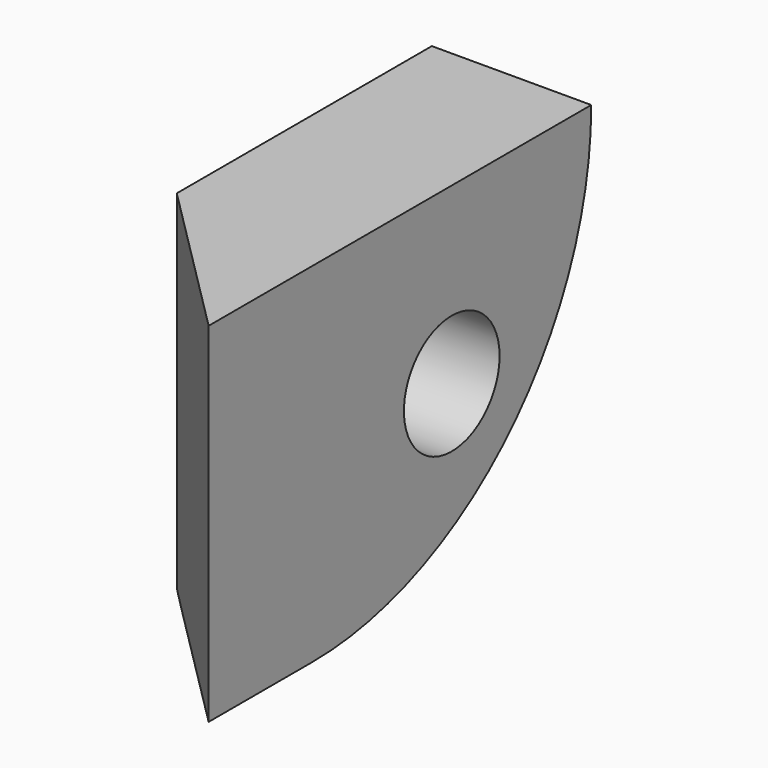
from build123d import *

# Parameters (mm, degrees)
F0_W     = 76.2
F0_H     = 55.5625
F1_DEPTH = 25.4
F2_R     = 55.56249
F3_R     = 9.525
F4_DEPTH = 25.4
F6_DEPTH = 55.5635


# Not quite as in the source:
# - a fillet or chamfer is up to 0.001 mm smaller than in the source, because OpenCascade refuses the exact size


with BuildPart() as f1:
    # F0 (on Right) → F1 (new body)
    with BuildSketch(Plane.YZ):
        Rectangle(F0_W, F0_H)
    extrude(amount=F1_DEPTH)

    # F2 (radius 55.5625 in the source; OpenCascade refuses exactly that, so slightly less here)
    f2_edges = [f1.edges().sort_by_distance(p)[0] for p in [
        (12.7, 38.1, -27.78125),
    ]]
    fillet(f2_edges, radius=F2_R)

    # F3 (on face) → F4 (cut)
    with BuildSketch(Plane.YZ.offset(25.4)):
        with Locations((10.31875, 0)):
            Circle(F3_R)
    extrude(amount=-F4_DEPTH, mode=Mode.SUBTRACT)

    # F5 (on face) → F6 (cut, through all)
    with BuildSketch(Plane.XY.offset(27.78125)):
        Polygon((0, -38.1), (25.4, -38.1), (0, -12.7), align=None)
    extrude(amount=-F6_DEPTH, mode=Mode.SUBTRACT)


solid = f1.part
